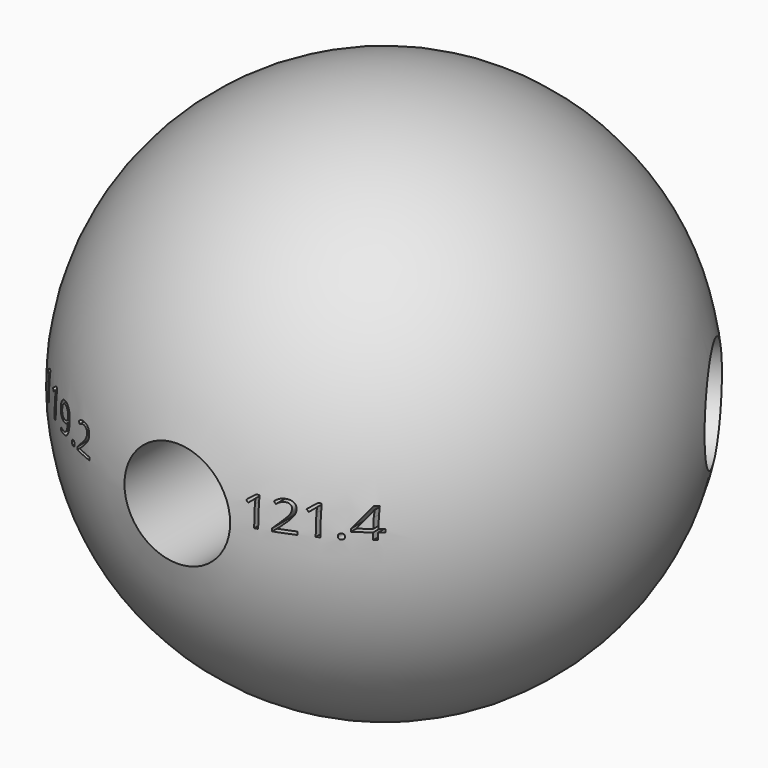
from build123d import *

# Parameters (mm, degrees)
F4_R           = 3.175
F5_DEPTH       = 25.4
F6_ANGLE       = -119.2
F7_ANGLE       = -119.5
F9_TEXT_SIZE   = 2.3646812123
F9_TEXT_SIZE_2 = 2.457870869
F10_DEPTH      = 8.9662
F12_TEXT_SIZE  = 3.130745285
F13_DEPTH      = 9.2456


# Not quite as in the source:
# - Text() gives the source's letters only with a copy of the font that has no kerning and outlines rounded to 1/6400 em; it was checked with that copy


with BuildPart() as f1:
    # F0 (on Top) → F1 (revolve)
    with BuildSketch(Plane.XY):
        with BuildLine():
            Line((0, -15.875), (0, 15.875))
            ThreePointArc((0, 15.875), (-15.875, 0), (0, -15.875))
        make_face()
    revolve(axis=Axis((0, 0, 0), (0, -1, 0)))

    # F9 (on offset) → F10 (cut)
    with BuildSketch(Plane.XZ.offset(19.05)):
        with Locations((-11.8693513796, 0)):
            Text('119.2', F9_TEXT_SIZE, font='Open Sans', text_align=(TextAlign.LEFT, TextAlign.BOTTOM))
        with Locations((3.7199493963, 0)):
            Text('121.4', F9_TEXT_SIZE_2, font='Open Sans', text_align=(TextAlign.LEFT, TextAlign.BOTTOM))
    extrude(amount=-F10_DEPTH, mode=Mode.SUBTRACT)

    # F12 (on offset) → F13 (cut)
    with BuildSketch(Plane(origin=(16.277440714, 9.8968390813, 0), x_dir=(-0.5195191119, 0.8544588301, 0), z_dir=(0.8544588301, 0.5195191119, 0))):
        with Locations((3.561118152, 0)):
            Text('119.5', F12_TEXT_SIZE, font='Open Sans', text_align=(TextAlign.LEFT, TextAlign.BOTTOM))
    extrude(amount=-F13_DEPTH, mode=Mode.SUBTRACT)


with BuildPart() as f5:
    # F4 (on offset) → F5 (new body)
    with BuildSketch(Plane.XZ.offset(6.35)):
        Circle(F4_R)
    extrude(amount=F5_DEPTH)


with BuildPart() as f6_1:
    # F6: copy of F5
    add(f5.part.rotate(Axis((0, 0, 28.4007303417), (0, 0, 1)), F6_ANGLE))


with BuildPart() as f7_1:
    # F7: copy of F6_1
    add(f6_1.part.rotate(Axis((0, 0, 28.4007303417), (0, 0, 1)), F7_ANGLE))


with BuildPart() as f1_1:
    add(f1.part)

    # F14: cut F6_1, F5, F7_1
    add(f6_1.part, mode=Mode.SUBTRACT)
    add(f5.part, mode=Mode.SUBTRACT)
    add(f7_1.part, mode=Mode.SUBTRACT)


solid = f1_1.part
